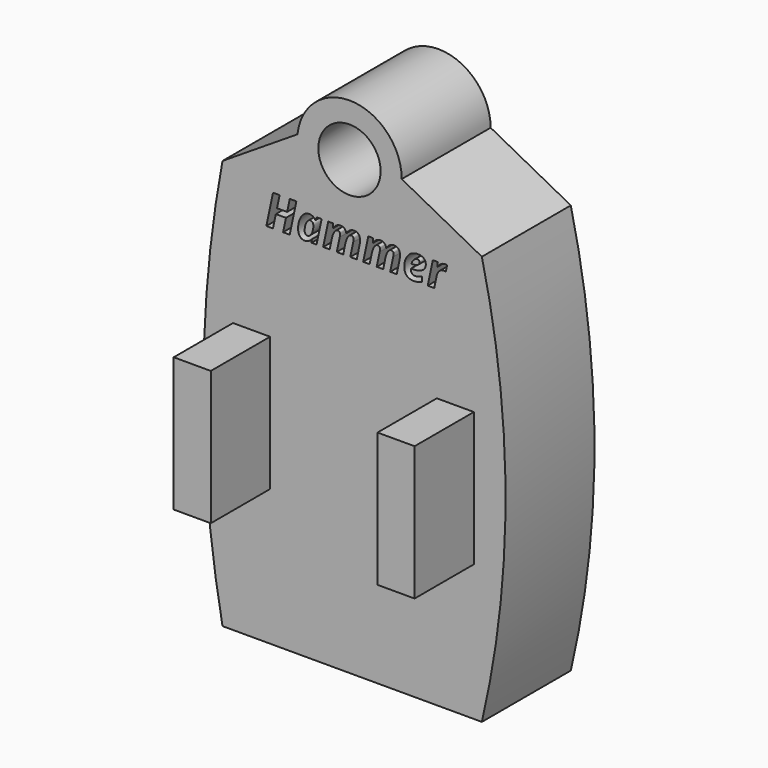
from build123d import *

# Parameters (mm, degrees)
F0_R         = 8.4012944475
F1_DEPTH     = 30
F2_W         = 10
F2_H         = 36.190473377
F3_DEPTH     = 50
F4_TEXT_SIZE = 11.9202640942
F5_DEPTH     = 50


# Not quite as in the source:
# - Text() gives the source's letters only with a copy of the font that has no kerning and outlines rounded to 1/6400 em; it was checked with that copy


with BuildPart() as f1:
    # F0 (on Front) → F1 (new body)
    with BuildSketch(Plane.XZ):
        with BuildLine():
            ThreePointArc((-23.4281154497, 40.6627374504), (-28.5880567377, -14.6004203193), (-23.4281154497, -69.8635780891))
            Line((-23.4281154497, -69.8635780891), (46.5718845503, -69.8635780891))
            ThreePointArc((46.5718845503, -69.8635780891), (52.958605845, -14.6004203193), (46.5718845503, 40.6627374504))
            Line((46.5718845503, 40.6627374504), (24.9412866608, 52.0837901195))
            ThreePointArc((24.9412866608, 52.0837901195), (11.5746761438, 66.1706313765), (-3.1936411689, 53.5610248377))
            Line((-3.1936411689, 53.5610248377), (-23.4281154497, 40.6627374504))
        make_face()
        with Locations((10.8350413702, 52.0837901195)):
            Circle(F0_R, mode=Mode.SUBTRACT)
    extrude(amount=F1_DEPTH)

    # F2 (on Front) → F3 (join)
    with BuildSketch(Plane.XZ):
        with Locations((-15.5880567377, -15.0275244378)):
            Rectangle(F2_W, F2_H)
        with Locations((39.4119432623, -15.0275244378)):
            Rectangle(F2_W, F2_H)
    extrude(amount=F3_DEPTH)

    # F4 (on Front) → F5 (cut)
    with BuildSketch(Plane.XZ):
        with Locations((-11.9001707062, 29.0375631303)):
            Text('Hammer', F4_TEXT_SIZE, font='Open Sans', font_style=FontStyle.BOLDITALIC, text_align=(TextAlign.LEFT, TextAlign.BOTTOM))
    extrude(amount=F5_DEPTH, mode=Mode.SUBTRACT)


solid = f1.part
